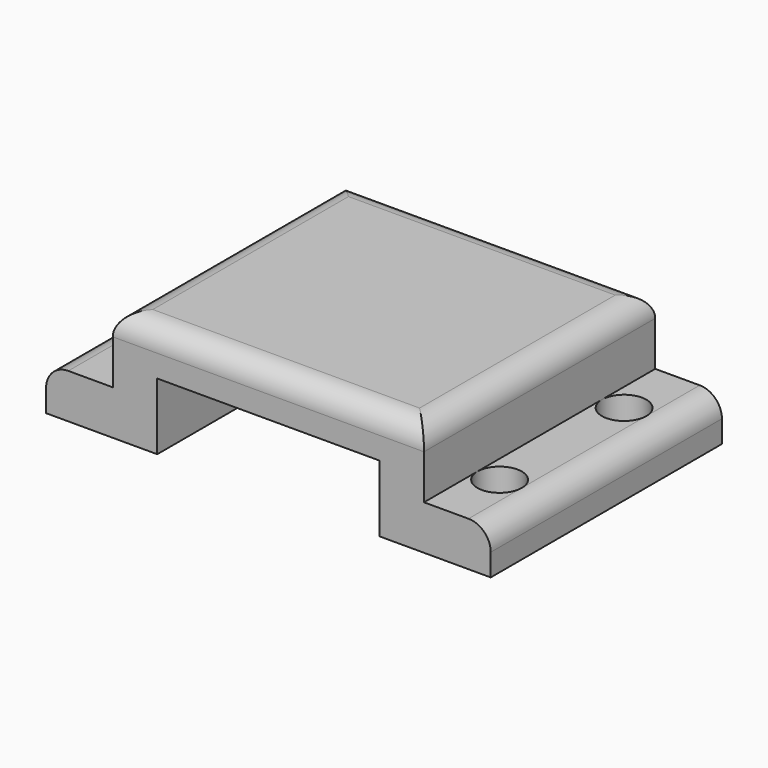
from build123d import *

# Parameters (mm, degrees)
F1_DEPTH = 13
F2_R     = 1
F3_R     = 1
F4_DEPTH = 25
F5_R     = 1
F6_DEPTH = 25


with BuildPart() as f1:
    # F0 (on Front) → F1 (new body)
    with BuildSketch(Plane.XZ):
        Polygon((-20.602078989, 0), (-18.61380395, 0), (-15.602078989, 0), (-15.602078989, 3), (-5.602078989, 3), (-5.602078989, 0), (-0.602078989, 0), (-0.602078989, 2), (-3.602078989, 2), (-3.602078989, 5), (-17.602078989, 5), (-17.602078989, 2), (-20.602078989, 2), align=None)
    extrude(amount=F1_DEPTH)

    # F2
    f2_edges = [f1.edges().sort_by_distance(p)[0] for p in [
        (-10.602079, 0, 5),
        (-3.602079, -6.5, 5),
        (-17.602079, -6.5, 5),
        (-10.602079, -13, 5),
        (-0.602079, -6.5, 2),
        (-20.602079, -6.5, 2),
    ]]
    fillet(f2_edges, radius=F2_R)

    # F3 (on face) → F4 (cut)
    with BuildSketch(Plane(origin=(0, 0, 0), x_dir=(1, 0, 0), z_dir=(0, 0, -1))):
        with Locations((-18.602078989, 10)):
            Circle(F3_R)
        with Locations((-18.602078989, 3)):
            Circle(F3_R)
    extrude(amount=-F4_DEPTH, mode=Mode.SUBTRACT)

    # F5 (on face) → F6 (cut)
    with BuildSketch(Plane(origin=(0, 0, 0), x_dir=(1, 0, 0), z_dir=(0, 0, -1))):
        with Locations((-2.602078989, 10)):
            Circle(F5_R)
        with Locations((-2.602078989, 3)):
            Circle(F5_R)
    extrude(amount=-F6_DEPTH, mode=Mode.SUBTRACT)


solid = f1.part
